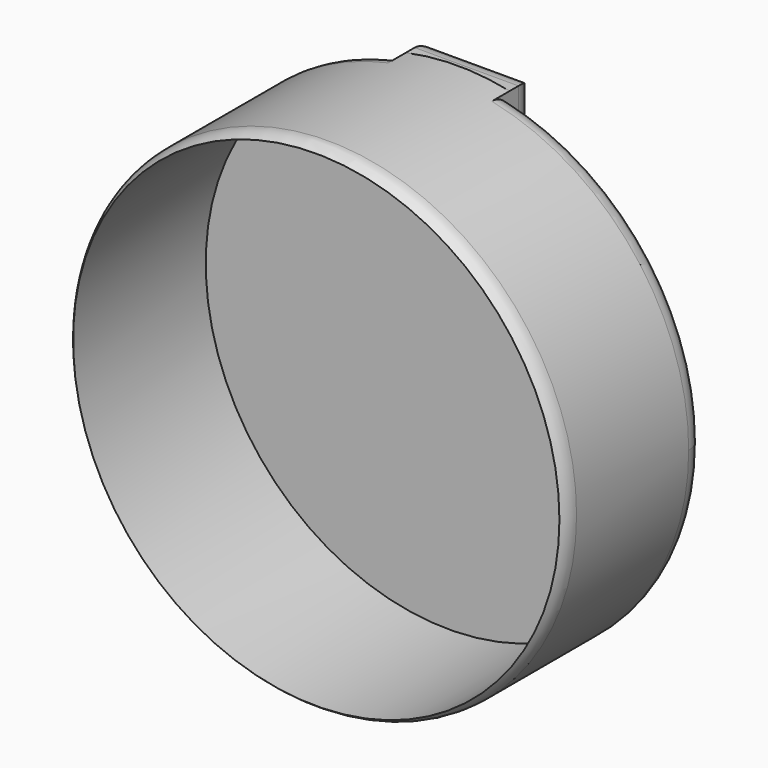
from build123d import *

# Parameters (mm, degrees)
F0_R         = 11.2475
F1_DEPTH     = 8
F2_R         = 11
F3_DEPTH     = 7.5
F4_W         = 4.6930826756
F4_H         = 22
F5_DEPTH     = 1.5
F6_T1_DEPTH  = 9.6930826756
F6_T3_DEPTH  = 27
F6_T8_ANGLE  = 90.6971129065
F6_T13_ANGLE = 181.4172742502
F6_T18_ANGLE = 90.6971129065


# Not quite as in the source:
# - a fillet or chamfer that OpenCascade refuses, or shapes differently, is made with other operations: its cross-section is extruded or revolved along the edge and cut away or added


with BuildPart() as f1:
    # F0 (on Front) → F1 (new body)
    with BuildSketch(Plane.XZ):
        Circle(F0_R)
    extrude(amount=F1_DEPTH)

    # F2 (on face) → F3 (cut)
    with BuildSketch(Plane.XZ.offset(8)):
        Circle(F2_R)
    extrude(amount=-F3_DEPTH, mode=Mode.SUBTRACT)

    # F4 (on face) → F5 (join)
    with BuildSketch(Plane(origin=(0, 0, 0), x_dir=(-1, 0, 0), z_dir=(0, 1, 0))):
        Rectangle(F4_W, F4_H)
    extrude(amount=F5_DEPTH)

    # F6: fillet of radius 1 on 9 edges, made by hand

    # F6_s2 → F6_t1 (cut)
    with BuildSketch(Plane.YZ.offset(-4.8465413378)):
        with BuildLine():
            ThreePointArc((0.5, -11), (1.2071067812, -10.7071067812), (1.5, -10))
            Line((1.5, -10), (1.5, -11))
            Line((1.5, -11), (0.5, -11))
        make_face()
        with BuildLine():
            ThreePointArc((0.5, 11), (1.2071067812, 10.7071067812), (1.5, 10))
            Line((1.5, 10), (1.5, 11))
            Line((1.5, 11), (0.5, 11))
        make_face()
    extrude(amount=F6_T1_DEPTH, mode=Mode.SUBTRACT)

    # F6_s4 → F6_t3 (cut)
    with BuildSketch(Plane.XY.offset(-13.5)):
        with BuildLine():
            ThreePointArc((-2.3465413378, 0.5), (-2.053648119, 1.2071067812), (-1.3465413378, 1.5))
            Line((-1.3465413378, 1.5), (-2.3465413378, 1.5))
            Line((-2.3465413378, 1.5), (-2.3465413378, 0.5))
        make_face()
        with BuildLine():
            ThreePointArc((2.3465413378, 0.5), (2.053648119, 1.2071067812), (1.3465413378, 1.5))
            Line((1.3465413378, 1.5), (2.3465413378, 1.5))
            Line((2.3465413378, 1.5), (2.3465413378, 0.5))
        make_face()
    extrude(amount=F6_T3_DEPTH, mode=Mode.SUBTRACT)


with BuildPart() as f6_tool6:
    # F6_s7 → F6_t8 (revolve)
    with BuildSketch(Plane.XY):
        with BuildLine():
            ThreePointArc((11.2475, -1), (10.9546067812, -0.2928932188), (10.2475, 0))
            Line((10.2475, 0), (11.2475, 0))
            Line((11.2475, 0), (11.2475, -1))
        make_face()
    revolve(axis=Axis((0, 0, 0), (0, -1, 0)), revolution_arc=F6_T8_ANGLE)

    split(bisect_by=Plane.YZ.offset(2.3465413378), keep=Keep.TOP)


with BuildPart() as f1_1:
    add(f1.part)

    # F6_t5: cut F6_tool6
    add(f6_tool6.part, mode=Mode.SUBTRACT)


with BuildPart() as f6_tool11:
    # F6_s12 → F6_t13 (revolve)
    with BuildSketch(Plane(origin=(0, 0, 0), x_dir=(0, 1, 0), z_dir=(0.9999235166, 0, -0.0123677357))):
        with BuildLine():
            ThreePointArc((-1, 11.2475), (-0.2928932188, 10.9546067812), (0, 10.2475))
            Line((0, 10.2475), (0, 11.2475))
            Line((0, 11.2475), (-1, 11.2475))
        make_face()
    revolve(axis=Axis((0, 0, 0), (0, -1, 0)), revolution_arc=F6_T13_ANGLE)

    split(bisect_by=Plane.YZ.offset(-2.3465413378), keep=Keep.BOTTOM)


with BuildPart() as f1_2:
    add(f1_1.part)

    # F6_t10: cut F6_tool11
    add(f6_tool11.part, mode=Mode.SUBTRACT)


with BuildPart() as f6_tool16:
    # F6_s17 → F6_t18 (revolve)
    with BuildSketch(Plane(origin=(0, 0, 0), x_dir=(0, 1, 0), z_dir=(-0.999925984, 0, 0.0121666153))):
        with BuildLine():
            ThreePointArc((-1, 11.2475), (-0.2928932188, 10.9546067812), (0, 10.2475))
            Line((0, 10.2475), (0, 11.2475))
            Line((0, 11.2475), (-1, 11.2475))
        make_face()
    revolve(axis=Axis((0, 0, 0), (0, -1, 0)), revolution_arc=F6_T18_ANGLE)

    split(bisect_by=Plane.YZ.offset(2.3465413378), keep=Keep.TOP)


with BuildPart() as f1_3:
    add(f1_2.part)

    # F6_t15: cut F6_tool16
    add(f6_tool16.part, mode=Mode.SUBTRACT)

    # F6_s20 → F6_t21 (revolve, cut)
    with BuildSketch(Plane.XY):
        with BuildLine():
            ThreePointArc((11.2475, -7.3414077513), (11.1835822613, -7.6931889333), (11, -8))
            Line((11, -8), (11.2475, -8))
            Line((11.2475, -8), (11.2475, -7.3414077513))
        make_face()
    revolve(axis=Axis((0, -8, 0), (0, -1, 0)), mode=Mode.SUBTRACT)


solid = f1_3.part
